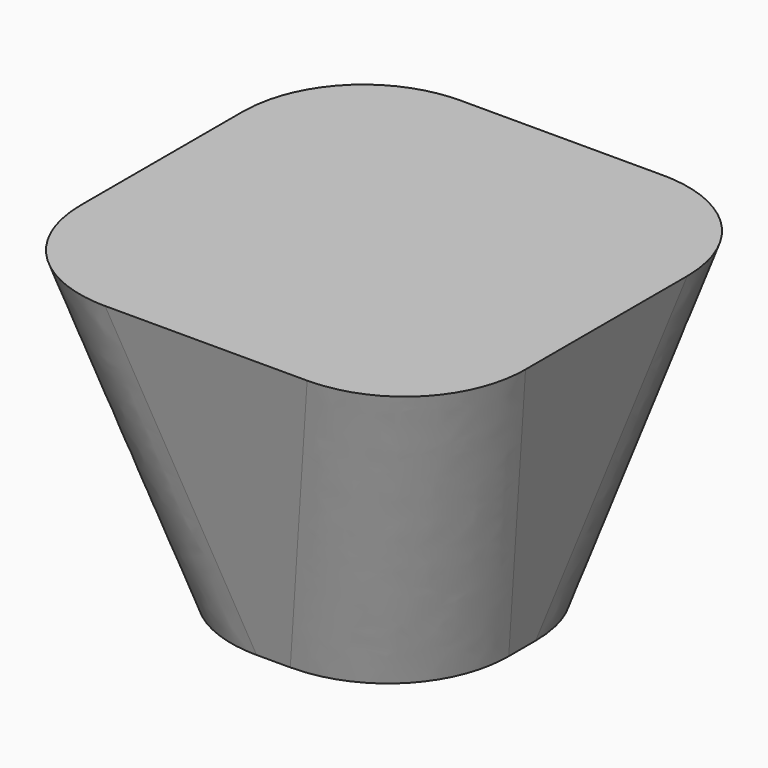
from build123d import *

# Parameters (mm, degrees)
F0_W     = 22
F0_H     = 22
F1_DEPTH = 25
F1_TAPER = -15
F2_R     = 10


with BuildPart() as f1:
    # F0 (on Top) → F1 (new body)
    with BuildSketch(Plane.XY):
        Rectangle(F0_W, F0_H)
    extrude(amount=F1_DEPTH, taper=F1_TAPER)

    # F2
    f2_edges = [f1.edges().sort_by_distance(p)[0] for p in [
        (-14.349365, -14.349365, 12.5),
        (-14.349365, 14.349365, 12.5),
        (14.349365, 14.349365, 12.5),
        (14.349365, -14.349365, 12.5),
    ]]
    fillet(f2_edges, radius=F2_R)


solid = f1.part
